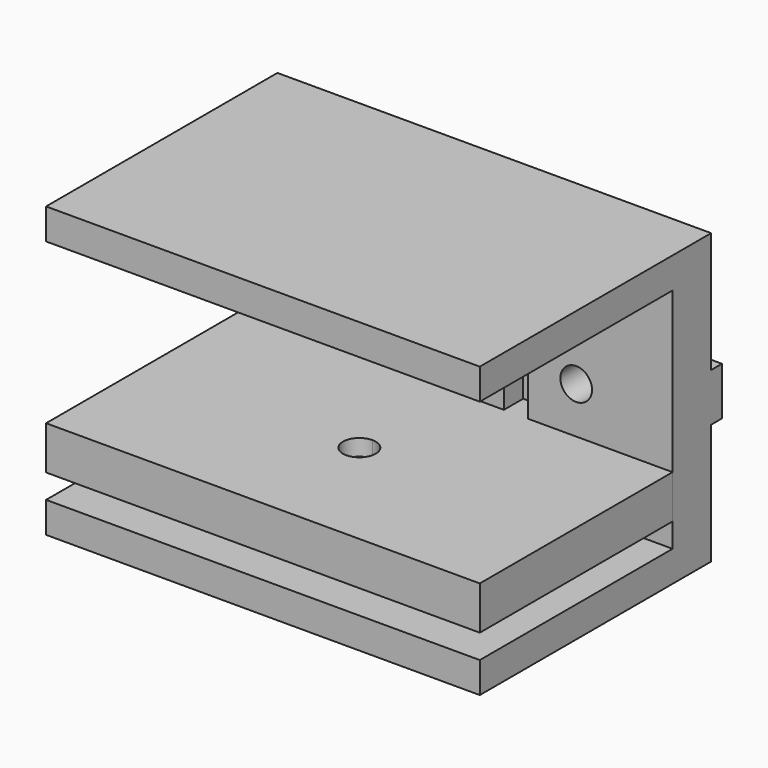
from build123d import *

# Parameters (mm, degrees)
F1_DEPTH = 114.3
F3_D     = 8.334375
F5_DEPTH = 12.7
F4_W     = 6.35
F4_H     = 6.35
F4_W_2   = 6.3500022411
F6_DEPTH = 55.88
F7_START = 6.35
F7_DEPTH = 11.43
F8_R     = 4.318
F9_DEPTH = 7.112


# Not quite as in the source:
# - a length typed as a fraction of an inch, garbled in the dataset ("3 / 203.2 mm" for 3/8 in), is restored


with BuildPart() as f1:
    # F0 (on Right) → F1 (new body)
    with BuildSketch(Plane.YZ):
        Polygon((-38.1, -29.972), (-38.1, -38.1), (38.1, -38.1), (38.1, -6.35), (41.656, -6.35), (41.656, 6.35), (38.1, 6.35), (38.1, 38.1), (-38.1, 38.1), (-38.1, 29.972), (25.4, 29.972), (25.4, 2.3702074885), (25.4, -29.972), align=None)
    extrude(amount=F1_DEPTH)

    # F3 (through all)
    with Locations(Plane.XZ.offset(-25.4)):
        with Locations((25.4, 0), (88.9, 0)):
            Hole(F3_D / 2)

    # F4 (on face) → F5 (cut)
    with BuildSketch(Plane.XY.offset(-29.972)):
        with BuildLine():
            ThreePointArc((57.1499993635, -2.032), (52.8319994397, -6.3500000762), (57.1499995159, -10.668))
            Line((57.1499995159, -10.668), (57.1499993635, -2.032))
        make_face()
        with BuildLine():
            Line((57.1499993635, -2.032), (57.1499995159, -10.668))
            ThreePointArc((57.1499995159, -10.668), (60.2032865478, -9.4032870542), (61.4679994397, -6.35))
            ThreePointArc((61.4679994397, -6.35), (60.2032864939, -3.2967128919), (57.1499993635, -2.032))
        make_face()
    extrude(amount=-F5_DEPTH, mode=Mode.SUBTRACT)

    # F4 (on face) → F6 (cut)
    with BuildSketch(Plane.XY.offset(-29.972)):
        with Locations((41.275, 28.575)):
            Rectangle(F4_W, F4_H)
        with Locations((73.0249988794, 28.575)):
            Rectangle(F4_W_2, F4_H)
    extrude(amount=F6_DEPTH, mode=Mode.SUBTRACT)


with BuildPart() as f7:
    # F4 (on face) → F7 (new body)
    with BuildSketch(Plane.XY.offset(-29.972).offset(F7_START)):
        with BuildLine():
            Line((0, -38.1), (57.15, -38.1))
            Line((57.15, -38.1), (57.1499995159, -10.668))
            ThreePointArc((57.1499995159, -10.668), (52.8319994397, -6.3500000762), (57.1499993635, -2.032))
            Line((57.1499993635, -2.032), (57.1499988794, 25.4))
            Line((57.1499988794, 25.4), (44.45, 25.4))
            Line((44.45, 25.4), (38.1, 25.4))
            Line((38.1, 25.4), (0, 25.4))
            Line((0, 25.4), (0, -38.1))
        make_face()
        with Locations((41.275, 28.575)):
            Rectangle(F4_W, F4_H)
        with Locations((73.0249988794, 28.575)):
            Rectangle(F4_W_2, F4_H)
        with BuildLine():
            Line((114.3, -38.1), (114.3, 25.4))
            Line((114.3, 25.4), (76.2, 25.4))
            Line((76.2, 25.4), (69.8499977589, 25.4))
            Line((69.8499977589, 25.4), (57.1499988794, 25.4))
            Line((57.1499988794, 25.4), (57.1499993635, -2.032))
            ThreePointArc((57.1499993635, -2.032), (60.2032864939, -3.2967128919), (61.4679994397, -6.35))
            ThreePointArc((61.4679994397, -6.35), (60.2032865478, -9.4032870542), (57.1499995159, -10.668))
            Line((57.1499995159, -10.668), (57.15, -38.1))
            Line((57.15, -38.1), (114.3, -38.1))
        make_face()
    extrude(amount=F7_DEPTH)

    # F8 (on face) → F9 (cut)
    with BuildSketch(Plane(origin=(0, 0, -23.622), x_dir=(1, 0, 0), z_dir=(0, 0, -1))):
        Polygon((60.2179755791, 13.0096438149), (52.9165667855, 12.3367671824), (49.8485906462, 5.6771233675), (54.0820233003, -0.3096438149), (61.3834320939, 0.3632328176), (64.4514082333, 7.0228766325), align=None)
        with Locations((57.1499994397, 6.35)):
            Circle(F8_R, mode=Mode.SUBTRACT)
    extrude(amount=-F9_DEPTH, mode=Mode.SUBTRACT)


solid = Compound([f1.part, f7.part])
